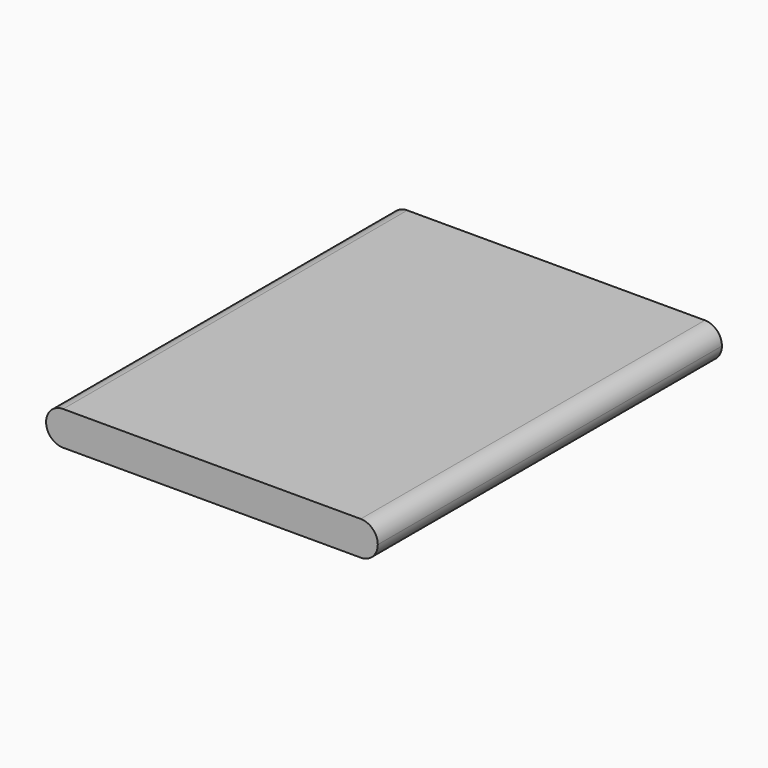
from build123d import *

# Parameters (mm, degrees)
F0_W     = 42.0116
F0_H     = 54.483
F1_DEPTH = 4.318
F2_R     = 2.15899


# Not quite as in the source:
# - a fillet or chamfer is up to 0.001 mm smaller than in the source, because OpenCascade refuses the exact size


with BuildPart() as f1:
    # F0 (on Top) → F1 (new body)
    with BuildSketch(Plane.XY):
        with Locations((-5.6643610103, -14.8812746114)):
            Rectangle(F0_W, F0_H)
    extrude(amount=F1_DEPTH)

    # F2 (radius 2.159 in the source; OpenCascade refuses exactly that, so slightly less here)
    f2_edges = [f1.edges().sort_by_distance(p)[0] for p in [
        (-26.670161, -14.881275, 4.318),
        (15.341439, -14.881275, 4.318),
        (-26.670161, -14.881275, 0),
        (15.341439, -14.881275, 0),
    ]]
    fillet(f2_edges, radius=F2_R)


solid = f1.part
